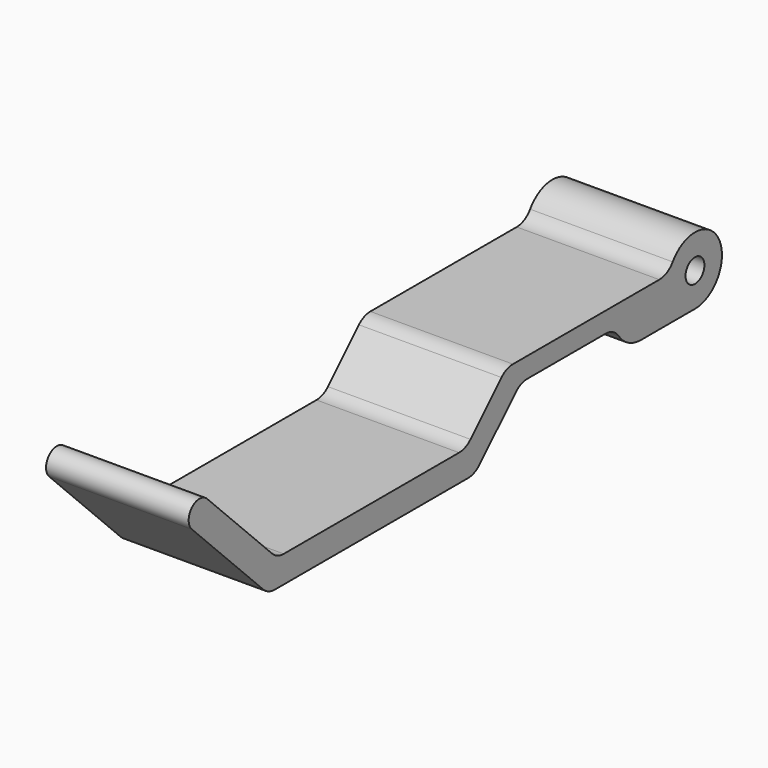
from build123d import *

# Parameters (mm, degrees)
F0_R          = 1.75
F1_DEPTH      = 15.875
F3_DEPTH      = 31.75
F4_R          = 3
F5_W          = 5
F5_H          = 35
F6_DEPTH      = 10.001
F6_DEPTH_BACK = 7.5573491861
F7_T1_DEPTH   = 8.7055800262
F7_T3_DEPTH   = 8.75
F7_T5_DEPTH   = 8.75
F7_T7_DEPTH   = 8.7055800262
F8_DEPTH      = 0.3
F9_DEPTH      = 0.3
F10_DEPTH     = 5.3
F11_DEPTH     = 5.3


# Not quite as in the source:
# - a fillet or chamfer that OpenCascade refuses, or shapes differently, is made with other operations: its cross-section is extruded or revolved along the edge and cut away or added


with BuildPart() as f1:
    # F0 (on Right) → F1 (new body, symmetric)
    with BuildSketch(Plane.YZ):
        with BuildLine():
            Line((-5.2303039929, -1.5), (-4.7696960071, -1.5))
            ThreePointArc((-4.7696960071, -1.5), (5, 0), (-4.7696960071, 1.5))
            Line((-4.7696960071, 1.5), (-35, 1.5))
            Line((-35, 1.5), (-42.5, -6))
            Line((-42.5, -6), (-77.5, -6))
            Line((-77.5, -6), (-90.4705627485, 6.9705627485))
            ThreePointArc((-90.4705627485, 6.9705627485), (-93.2989898732, 6.9705627485), (-93.2989898732, 4.1421356237))
            Line((-93.2989898732, 4.1421356237), (-79.1568542495, -10))
            Line((-79.1568542495, -10), (-40.8431457505, -10))
            Line((-40.8431457505, -10), (-32.3431457505, -1.5))
            Line((-32.3431457505, -1.5), (-14.7696960071, -1.5))
            ThreePointArc((-14.7696960071, -1.5), (-10, -5), (-5.2303039929, -1.5))
        make_face()
        Circle(F0_R, mode=Mode.SUBTRACT)
    extrude(amount=F1_DEPTH, both=True)

    # F2 (on face) → F3 (join, through all)
    with BuildSketch(Plane.YZ.offset(15.875)):
        with BuildLine():
            ThreePointArc((-5.2303039929, -1.5), (-7.0419601085, -4.0311288741), (-10, -5))
            Line((-10, -5), (0, -5))
            ThreePointArc((0, -5), (-2.9580398915, -4.0311288741), (-4.7696960071, -1.5))
            Line((-4.7696960071, -1.5), (-5.2303039929, -1.5))
        make_face()
    extrude(amount=-F3_DEPTH)

    # F4
    f4_edges = [f1.edges().sort_by_distance(p)[0] for p in [
        (0, -4.769696, 1.5),
        (0, -14.769696, -1.5),
        (0, -77.5, -6),
        (0, -79.156854, -10),
        (0, -40.843146, -10),
        (0, -32.343146, -1.5),
        (0, -42.5, -6),
        (0, -35, 1.5),
    ]]
    fillet(f4_edges, radius=F4_R)

    # F5 (on Top) → F6 (cut, two sides)
    with BuildSketch(Plane.XY) as f6_sk:
        with Locations((-13.375, -12.5)):
            Rectangle(F5_W, F5_H)
        with Locations((13.375, -12.5)):
            Rectangle(F5_W, F5_H)
    extrude(amount=-F6_DEPTH, mode=Mode.SUBTRACT)
    extrude(f6_sk.sketch, amount=F6_DEPTH_BACK, mode=Mode.SUBTRACT)

    # F7: fillet of radius 1.5 on 4 edges, made by hand

    # F7_s2 → F7_t1 (cut)
    with BuildSketch(Plane.YZ.offset(10.875)):
        with BuildLine():
            ThreePointArc((-31.3668350211, -1.5118453264), (-30.3932598615, -1.0302531824), (-30, -0.0177679895))
            Line((-30, -0.0177679895), (-29.85, -0.0177679895))
            Line((-29.85, -0.0177679895), (-29.85, -1.5))
            Line((-29.85, -1.5), (-30, -1.65))
            ThreePointArc((-30, -1.65), (-31.1005050634, -1.65), (-31.3535185232, -1.66125306))
            Line((-31.3535185232, -1.66125306), (-31.3668350211, -1.5118453264))
        make_face()
    extrude(amount=F7_T1_DEPTH, mode=Mode.SUBTRACT)

    # F7_s4 → F7_t3 (cut)
    with BuildSketch(Plane.YZ.offset(10.875)):
        with BuildLine():
            ThreePointArc((-30, 0), (-30.4393398282, 1.0606601718), (-31.5, 1.5))
            Line((-31.5, 1.5), (-30, 1.5))
            Line((-30, 1.5), (-30, 0))
        make_face()
    extrude(amount=F7_T3_DEPTH, mode=Mode.SUBTRACT)

    # F7_s6 → F7_t5 (cut)
    with BuildSketch(Plane.YZ.offset(-19.625)):
        with BuildLine():
            ThreePointArc((-30, 0), (-30.4393398282, 1.0606601718), (-31.5, 1.5))
            Line((-31.5, 1.5), (-30, 1.5))
            Line((-30, 1.5), (-30, 0))
        make_face()
    extrude(amount=F7_T5_DEPTH, mode=Mode.SUBTRACT)

    # F7_s8 → F7_t7 (cut)
    with BuildSketch(Plane.YZ.offset(-19.5805800262)):
        with BuildLine():
            ThreePointArc((-31.3668350211, -1.5118453264), (-30.3932598615, -1.0302531824), (-30, -0.0177679895))
            Line((-30, -0.0177679895), (-29.85, -0.0177679895))
            Line((-29.85, -0.0177679895), (-29.85, -1.5))
            Line((-29.85, -1.5), (-30, -1.65))
            ThreePointArc((-30, -1.65), (-31.1005050634, -1.65), (-31.3535185232, -1.66125306))
            Line((-31.3535185232, -1.66125306), (-31.3668350211, -1.5118453264))
        make_face()
    extrude(amount=F7_T7_DEPTH, mode=Mode.SUBTRACT)

    # F8 (cut): a face of the model
    f8_faces = [f1.faces().sort_by_distance(p)[0] for p in [
        (10.875, -9.1101781633, -0.6280033564),
    ]]
    extrude(f8_faces, amount=-F8_DEPTH, mode=Mode.SUBTRACT)

    # F9 (cut): a face of the model
    f9_faces = [f1.faces().sort_by_distance(p)[0] for p in [
        (-10.875, -9.1101781633, -0.6280033564),
    ]]
    extrude(f9_faces, amount=-F9_DEPTH, mode=Mode.SUBTRACT)

    # F10 (cut, through all): a face of the model
    f10_faces = [f1.faces().sort_by_distance(p)[0] for p in [
        (15.875, -86.1987808312, -2.0211113015),
    ]]
    extrude(f10_faces, amount=-F10_DEPTH, mode=Mode.SUBTRACT)

    # F11 (cut, through all): a face of the model
    f11_faces = [f1.faces().sort_by_distance(p)[0] for p in [
        (-15.875, -86.1987808312, -2.0211113015),
    ]]
    extrude(f11_faces, amount=-F11_DEPTH, mode=Mode.SUBTRACT)


solid = f1.part
